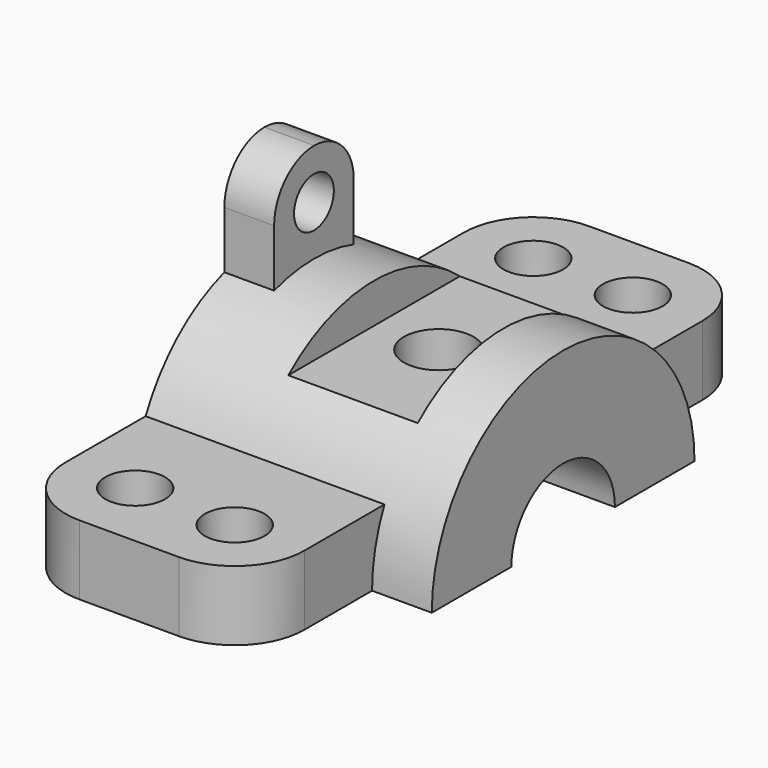
from build123d import *

# Parameters (mm, degrees)
F1_DEPTH  = 30
F2_R      = 6
F3_DEPTH  = 14
F4_R      = 5
F5_DEPTH  = 10
F7_W      = 26
F7_H      = 66
F8_DEPTH  = 8
F9_R      = 7
F10_DEPTH = 25.001


# Not quite as in the source:
# - a pattern or mirror of a feature is missing from the dataset's text; its kind, count and spacing are read off the source's solid


with BuildPart() as f1:
    # F0 (on Right) → F1 (new body, symmetric)
    with BuildSketch(Plane.YZ):
        with BuildLine():
            Line((13, 0), (33, 0))
            ThreePointArc((33, 0), (0, 33), (-33, 0))
            Line((-33, 0), (-13, 0))
            ThreePointArc((-13, 0), (0, 13), (13, 0))
        make_face()
    extrude(amount=F1_DEPTH, both=True)

    # F2 (on face) → F3 (join)
    with BuildSketch(Plane(origin=(0, 0, 0), x_dir=(1, 0, 0), z_dir=(0, 0, -1))):
        with BuildLine():
            Line((18, 28.1032323837), (18, 33))
            Line((18, 33), (18, 50))
            ThreePointArc((18, 50), (13.8994949366, 59.8994949366), (4, 64))
            Line((4, 64), (-16, 64))
            ThreePointArc((-16, 64), (-25.8994949366, 59.8994949366), (-30, 50))
            Line((-30, 50), (-30, 33))
            Line((-30, 33), (-30, 28.1032323837))
            Line((-30, 28.1032323837), (18, 28.1032323837))
        make_face()
        with Locations((-16, 50)):
            Circle(F2_R, mode=Mode.SUBTRACT)
        with Locations((4, 50)):
            Circle(F2_R, mode=Mode.SUBTRACT)
    f3 = extrude(amount=-F3_DEPTH)

    # F3_copies: F3 across plane
    add(f3.mirror(Plane.ZX))

    # F4 (on face) → F5 (join)
    with BuildSketch(Plane(origin=(-30, 0, 0), x_dir=(0, -1, 0), z_dir=(-1, 0, 0))):
        with BuildLine():
            ThreePointArc((10.1, 42.9), (7.1594782015, 50.0240348036), (0.0501243796, 52.9998756204))
            ThreePointArc((0.0501243796, 52.9998756204), (-6.9886795739, 50.0534120749), (-9.9, 43))
            Line((-9.9, 43), (-9.9, 30.9537276626))
            Line((-9.9, 30.9537276626), (10.1, 30.9537276626))
            Line((10.1, 30.9537276626), (10.1, 42.9))
        make_face()
        with Locations((0.1, 43)):
            Circle(F4_R, mode=Mode.SUBTRACT)
    extrude(amount=-F5_DEPTH)

    # F7 (on offset) → F8 (cut)
    with BuildSketch(Plane(origin=(0, 0, 33), x_dir=(1, 0, 0), z_dir=(0, 0, -1))):
        with Locations((5, 0)):
            Rectangle(F7_W, F7_H)
    extrude(amount=F8_DEPTH, mode=Mode.SUBTRACT)

    # F9 (on face) → F10 (cut, through all)
    with BuildSketch(Plane.XY.offset(25)):
        with Locations((5, 0)):
            Circle(F9_R)
    extrude(amount=-F10_DEPTH, mode=Mode.SUBTRACT)


with BuildPart() as f5:
    # F4 (on face) → F5, piece 2 (new body)
    with BuildSketch(Plane(origin=(-30, 0, 0), x_dir=(0, -1, 0), z_dir=(-1, 0, 0))):
        with BuildLine():
            Line((0.1, 53), (0, 53))
            ThreePointArc((0, 53), (0.025062267, 52.999968905), (0.0501243796, 52.9998756204))
            ThreePointArc((0.0501243796, 52.9998756204), (0.0750621123, 52.999968905), (0.1, 53))
        make_face()
    extrude(amount=-F5_DEPTH)


solid = Compound([f1.part, f5.part])
